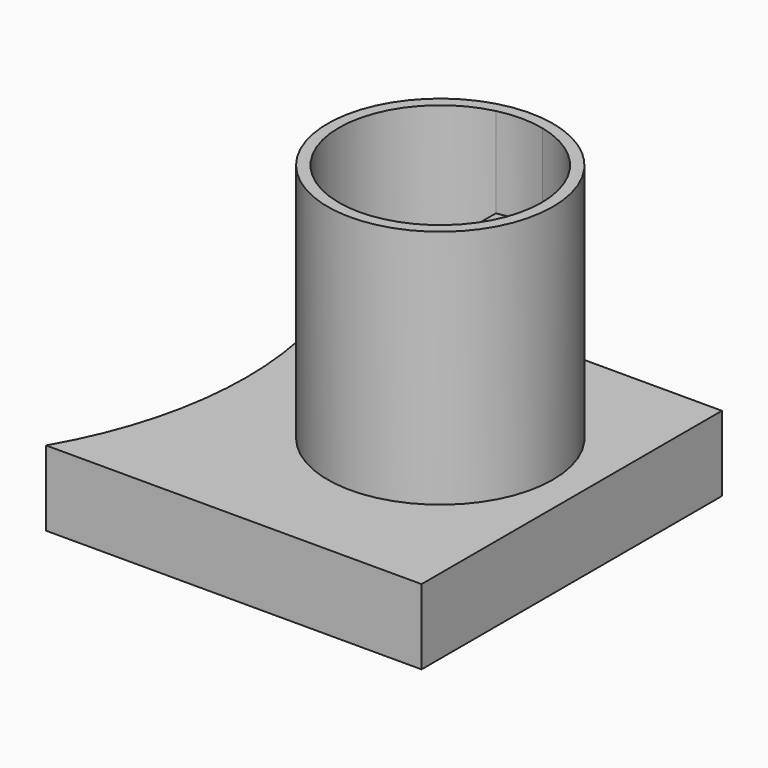
from build123d import *
from build123d import SkipClean  # not in build123d's __all__

# Parameters (mm, degrees)
F1_DEPTH = 10
F2_R     = 15
F3_DEPTH = 32
F4_DEPTH = 25
F5_DEPTH = 20


with BuildPart() as f1:
    # F0 (on Top) → F1 (new body)
    with BuildSketch(Plane.XY):
        with BuildLine():
            Line((-19.7133726581, 60.8366520235), (-69.7133726581, 60.8366520235))
            ThreePointArc((-69.7133726581, 60.8366520235), (-63.0146428473, 35.8366520235), (-69.7133726581, 10.8366520235))
            Line((-69.7133726581, 10.8366520235), (-19.7133726581, 10.8366520235))
            Line((-19.7133726581, 10.8366520235), (-19.7133726581, 60.8366520235))
        make_face()
    extrude(amount=F1_DEPTH)

    # F2 (on face) → F3 (join)
    with BuildSketch(Plane.XY.offset(10)):
        with Locations((-38.7318296711, 37.7283993232)):
            Circle(F2_R)
        with BuildLine():
            ThreePointArc((-35.6207755692, 50.8650405369), (-28.1429385494, 46.1024894119), (-25.2318296711, 37.7283993232))
            ThreePointArc((-25.2318296711, 37.7283993232), (-28.1429385494, 29.3543092346), (-35.6207755692, 24.5917581096))
            ThreePointArc((-35.6207755692, 24.5917581096), (-38.7318296711, 24.2283993232), (-41.8428837729, 24.5917581096))
            ThreePointArc((-41.8428837729, 24.5917581096), (-52.2318296711, 37.7283993232), (-41.8428837729, 50.8650405369))
            ThreePointArc((-41.8428837729, 50.8650405369), (-38.7318296711, 51.2283993232), (-35.6207755692, 50.8650405369))
        make_face(mode=Mode.SUBTRACT)
    extrude(amount=F3_DEPTH)

    # F2 (on face) → F4 (cut)
    with BuildSketch(Plane.XY.offset(10)):
        with BuildLine():
            Line((-41.8428837729, 24.5917581096), (-41.8428837729, 50.8650405369))
            ThreePointArc((-41.8428837729, 50.8650405369), (-52.2318296711, 37.7283993232), (-41.8428837729, 24.5917581096))
        make_face()
        with BuildLine():
            ThreePointArc((-35.6207755692, 24.5917581096), (-28.1429385494, 29.3543092346), (-25.2318296711, 37.7283993232))
            ThreePointArc((-25.2318296711, 37.7283993232), (-28.1429385494, 46.1024894119), (-35.6207755692, 50.8650405369))
            Line((-35.6207755692, 50.8650405369), (-35.6207755692, 24.5917581096))
        make_face()
    with SkipClean():  # cleaning this boolean's faces spoils the solid; the shape is the same uncleaned
        extrude(amount=-F4_DEPTH, mode=Mode.SUBTRACT)

    # F5 (add): a face of the model
    f5_faces = [f1.faces().sort_by_distance(p)[0] for p in [
        (-38.7318296711, 37.7283993232, 10),
    ]]
    with SkipClean():  # cleaning this boolean's faces spoils the solid; the shape is the same uncleaned
        extrude(f5_faces, amount=F5_DEPTH)


solid = f1.part
